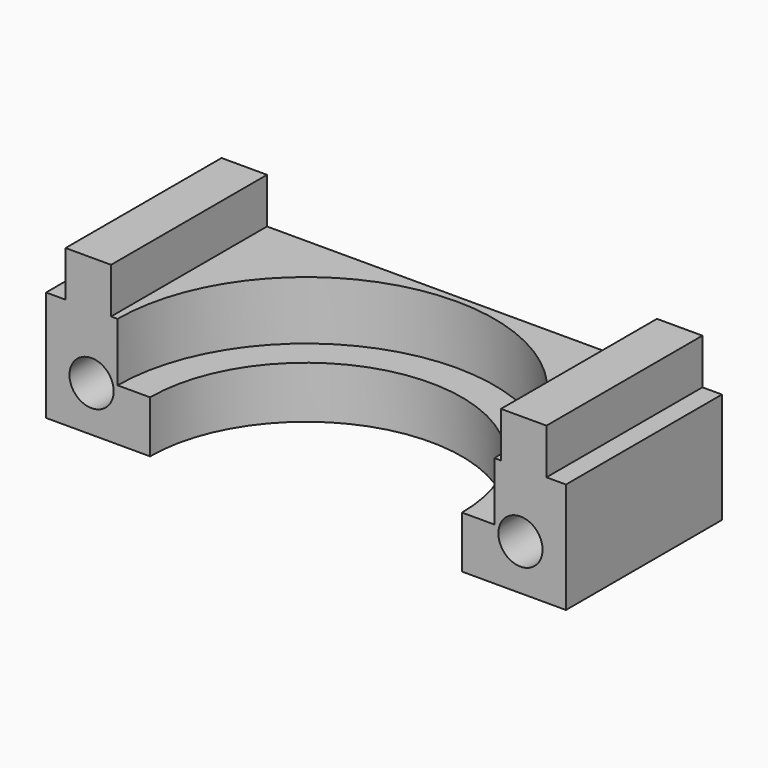
from build123d import *

# Parameters (mm, degrees)
F0_W            = 40
F0_H            = 15
F1_DEPTH        = 12
F3_DEPTH        = 8
F5_DEPTH        = 4
F6_W            = 1.5
F6_H            = 3.5
F7_DEPTH        = 15
F8_W            = 0.5
F8_H            = 3.5
F8_W_2          = 29.5
F9_DEPTH        = 15
F11_D           = 3.4
F11_CBORE_D     = 6.5
F11_CBORE_DEPTH = 3


# Not quite as in the source:
# - a pattern or mirror of a feature is missing from the dataset's text; its kind, count and spacing are read off the source's solid


with BuildPart() as f1:
    # F0 (on Top) → F1 (new body)
    with BuildSketch(Plane.XY):
        with Locations((0, -7.5)):
            Rectangle(F0_W, F0_H)
    extrude(amount=F1_DEPTH)

    # F2 (on face) → F3 (cut)
    with BuildSketch(Plane.XY.offset(12)):
        with BuildLine():
            Line((-14.5, -15), (14.5, -15))
            ThreePointArc((14.5, -15), (0, -0.5), (-14.5, -15))
        make_face()
    extrude(amount=-F3_DEPTH, mode=Mode.SUBTRACT)

    # F4 (on face) → F5 (cut, through all)
    with BuildSketch(Plane.XY.offset(4)):
        with BuildLine():
            Line((-12, -15), (12, -15))
            ThreePointArc((12, -15), (0, -3), (-12, -15))
        make_face()
    extrude(amount=-F5_DEPTH, mode=Mode.SUBTRACT)

    # F6 (on face) → F7 (cut, through all)
    with BuildSketch(Plane.XZ.offset(15)):
        with Locations((-19.25, 10.25)):
            Rectangle(F6_W, F6_H)
    f7 = extrude(amount=-F7_DEPTH, mode=Mode.SUBTRACT)

    # F7_copies: F7 across plane
    add(f7.mirror(Plane(origin=(0, 0, 0), x_dir=(0, 0, 1), z_dir=(1, 0, 0))), mode=Mode.SUBTRACT)

    # F8 (on face) → F9 (cut, through all)
    with BuildSketch(Plane.XZ.offset(15)):
        with Locations((-14.75, 10.25)):
            Rectangle(F8_W, F8_H)
        with Locations((0.25, 10.25)):
            Rectangle(F8_W_2, F8_H)
    extrude(amount=-F9_DEPTH, mode=Mode.SUBTRACT)

    # F11 (through all)
    with Locations(Plane(origin=(0, 0, 0), x_dir=(-1, 0, 0), z_dir=(0, 1, 0))):
        with Locations((-16.5, 3.5)):
            f11 = CounterBoreHole(F11_D / 2, F11_CBORE_D / 2, F11_CBORE_DEPTH)

    # F11_copies: F11 across plane
    add(f11.mirror(Plane(origin=(0, 0, 0), x_dir=(0, 0, -1), z_dir=(-1, 0, 0))), mode=Mode.SUBTRACT)


solid = f1.part
